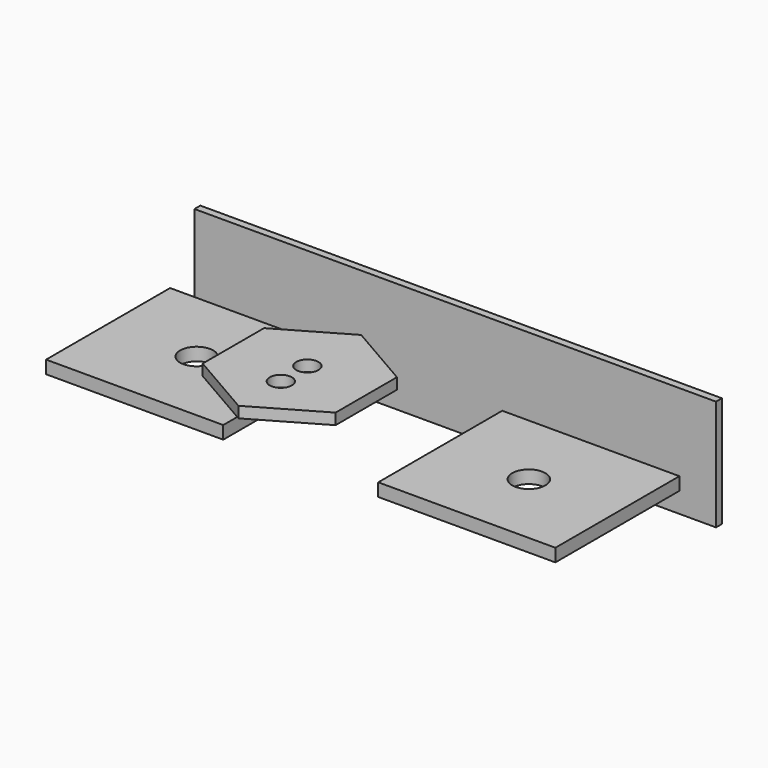
from build123d import *

# Parameters (mm, degrees)
F0_R          = 228.6
F0_W          = 545.1920032501
F0_H          = 1898.5517024994
F2_DEPTH      = 177.8
F0_W_2        = 1524
F0_H_2        = 711.2
F0_R_2        = 152.4
F4_DEPTH      = 1066.8
F5_DEPTH      = 914.4
F0_W_3        = 7178.9307594299
F0_H_3        = 101.6
F6_DEPTH      = 787.4
F6_DEPTH_BACK = 736.6


# Not quite as in the source:
# - the program builds the solid bodies; features that only make, move or delete a surface that nothing else refers to are left out


with BuildPart() as f2:
    # F0 (on Top) → F2 (new body)
    with BuildSketch(Plane.XY):
        Polygon((1219.2, 304.8), (1219.2, -484.2192232609), (1219.2, -997.4917173386), (1219.2, -1066.8), (3657.6, -1066.8), (3657.6, 1066.8), (1219.2, 1066.8), (1219.2, 914.4), align=None)
        with Locations((2438.4, 0)):
            Circle(F0_R, mode=Mode.SUBTRACT)
        with Locations((2988.1635904312, 5.0233006477)):
            Rectangle(F0_W, F0_H, mode=Mode.SUBTRACT)
        with Locations((2988.1635904312, 5.0233006477)):
            Rectangle(F0_W, F0_H)
    extrude(amount=F2_DEPTH)


with BuildPart() as f2b:
    # F0 (on Top) → F2, piece 2 (new body)
    with BuildSketch(Plane.XY):
        Polygon((-914.4, -1066.8), (-914.4, -364.223748142), (-914.4, 304.8), (-914.4, 914.4), (-914.4, 1066.8), (-3352.8, 1066.8), (-3352.8, -1066.8), align=None)
        with Locations((-2133.6, 0)):
            Circle(F0_R, mode=Mode.SUBTRACT)
        with Locations((-2186.1399059296, 679.8987394333)):
            Rectangle(F0_W_2, F0_H_2, mode=Mode.SUBTRACT)
        with Locations((-2186.1399059296, 679.8987394333)):
            Rectangle(F0_W_2, F0_H_2)
    extrude(amount=F2_DEPTH)


with BuildPart() as f4:
    # F0 (on Top) → F4 (new body)
    with BuildSketch(Plane.XY):
        Polygon((914.4, -364.223748142), (0, 163.705338005), (-914.4, -364.223748142), (-914.4, -1066.8), (-914.4, -1420.081920436), (0, -1948.011006583), (914.4, -1420.081920436), (914.4, -997.4917173386), (914.4, -484.2192232609), align=None)
        with Locations((0, -1219.2)):
            Circle(F0_R_2, mode=Mode.SUBTRACT)
        with Locations((0, -762)):
            Circle(F0_R_2, mode=Mode.SUBTRACT)
    extrude(amount=F4_DEPTH)

    # F0 (on Top) → F5 (cut)
    with BuildSketch(Plane.XY):
        Polygon((914.4, -364.223748142), (0, 163.705338005), (-914.4, -364.223748142), (-914.4, -1066.8), (-914.4, -1420.081920436), (0, -1948.011006583), (914.4, -1420.081920436), (914.4, -997.4917173386), (914.4, -484.2192232609), align=None)
        with Locations((0, -1219.2)):
            Circle(F0_R_2, mode=Mode.SUBTRACT)
        with Locations((0, -762)):
            Circle(F0_R_2, mode=Mode.SUBTRACT)
    extrude(amount=F5_DEPTH, mode=Mode.SUBTRACT)


with BuildPart() as f6:
    # F0 (on Top) → F6 (new body, two sides)
    with BuildSketch(Plane.XY) as f6_sk:
        with Locations((23.4687328339, 1803.4)):
            Rectangle(F0_W_3, F0_H_3)
    extrude(amount=F6_DEPTH)
    extrude(f6_sk.sketch, amount=-F6_DEPTH_BACK)


solid = Compound([f2.part, f2b.part, f4.part, f6.part])
